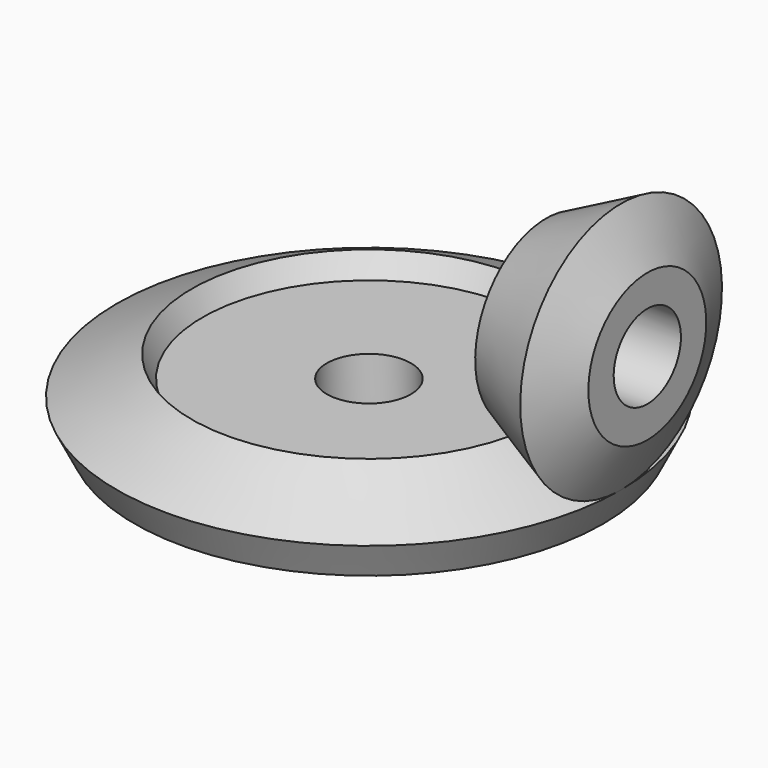
from build123d import *


# Not quite as in the source:
# - ends of sketch curves that miss each other by under 0.0002 mm in the source are joined


with BuildPart() as f2:
    # F1 (on Front) → F2 (revolve)
    with BuildSketch(Plane.XZ):
        Polygon((10.5357933703, 3.3501373036), (9.8931459258, 2.0648424145), (2.5, 2.0648456312), (2.5, -1), (13.9409830056, -1), (15, 1.1180339887), align=None)
    revolve(axis=Axis((0, 0, 3.0726052355), (0, 0, -1)))

    # F4 (on Front) → F5 (revolve)
    with BuildSketch(Plane.XZ):
        Polygon((11.4284392065, 6.1180339887), (11.4284392065, 5.135428976), (10.5357933703, 3.3501373036), (15, 1.1180339887), (16.5590169944, 4.2360679775), (16.5590169944, 6.1180339887), align=None)
    revolve(axis=Axis((9.5441560864, 0, 8.6180339887), (1, 0, 0)))


solid = f2.part
